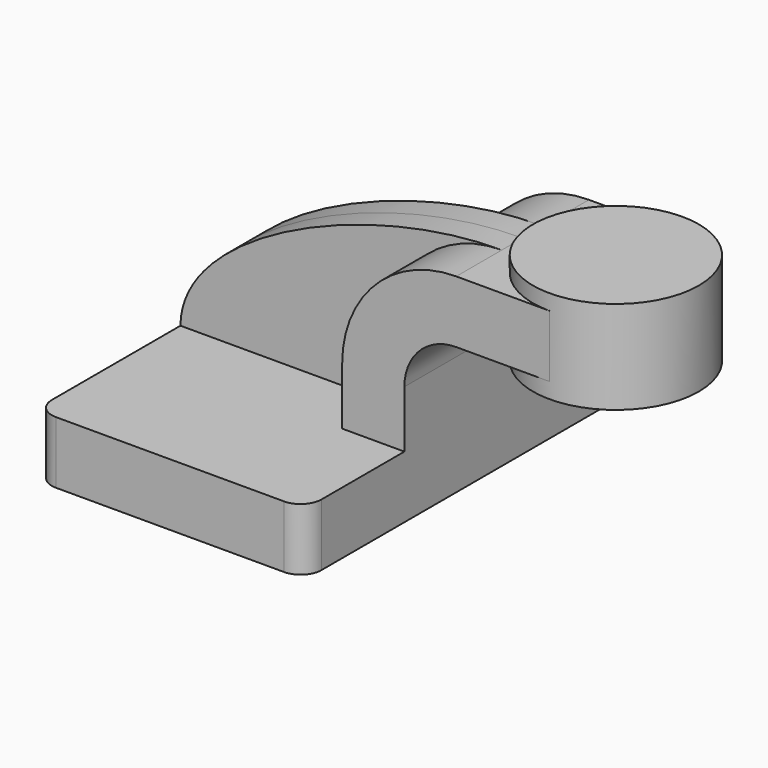
from build123d import *

# Parameters (mm, degrees)
F1_DEPTH = 63.5
F2_DEPTH = 25.4
F3_DEPTH = 7.9375
F0_W     = 25.4
F0_H     = 19.0500000358
F4_DEPTH = 25.4
F6_R     = 6.35


# Not quite as in the source:
# - a feature names something its author has since deleted; it is built from what else it names


with BuildPart() as f1:
    # F0 (on Front) → F1 (new body, symmetric)
    with BuildSketch(Plane.XZ):
        Polygon((-41.275, 9.525), (-41.275, -9.525), (41.275, -9.525), (41.275, 9.525), (22.2249999642, 9.525), align=None)
    extrude(amount=F1_DEPTH, both=True)

    # F0 (on Front) → F2 (join, symmetric)
    with BuildSketch(Plane.XZ):
        with BuildLine():
            Line((22.2249999642, 9.525), (41.275, 9.525))
            Line((41.275, 9.525), (41.275, 27.0002))
            ThreePointArc((41.275, 27.0002), (45.9246798487, 38.2255201513), (57.15, 42.8752))
            Line((57.15, 42.8752), (60.325, 42.8752))
            Line((60.325, 42.8752), (60.325, 61.9252000358))
            Line((60.325, 61.9252000358), (57.15, 61.9252000358))
            ThreePointArc((57.15, 61.9252000358), (32.4542956418, 51.6959043582), (22.2249999642, 27.0002))
            Line((22.2249999642, 27.0002), (22.2249999642, 9.525))
        make_face()
    extrude(amount=F2_DEPTH, both=True)

    # F0 (on Front) → F3 (join, symmetric)
    with BuildSketch(Plane.XZ):
        with BuildLine():
            add(Edge.make_bspline(
                [(-41.275, 9.525), (-41.1172062159, 36.9034484029), (15.5369872227, 62.0494298637), (57.15, 61.9252000358)],
                knots=[0, 0, 0, 0, 111.5045361803, 111.5045361803, 111.5045361803, 111.5045361803], degree=3))
            Line((-41.275, 9.525), (22.2249999642, 9.525))
            Line((22.2249999642, 9.525), (22.2249999642, 27.0002))
            ThreePointArc((22.2249999642, 27.0002), (32.4542956418, 51.6959043582), (57.15, 61.9252000358))
        make_face()
    extrude(amount=F3_DEPTH, both=True)

    # F0 (on Front) → F4 (join, symmetric)
    with BuildSketch(Plane.XZ):
        with Locations((73.025, 52.4002000179)):
            Rectangle(F0_W, F0_H)
    extrude(amount=F4_DEPTH, both=True)

    # F0 (on Front) → F5 (revolve)
    with BuildSketch(Plane.XZ):
        Polygon((85.725, 66.675), (85.725, 61.9252000358), (85.725, 42.8752), (85.725, 38.1), (111.125, 38.1), (111.125, 66.675), align=None)
    revolve(axis=Axis((85.725, 0, 52.3875), (0, 0, 1)))

    # F6
    f6_edges = [f1.edges().sort_by_distance(p)[0] for p in [
        (41.275, -63.5, 0),
        (-41.275, -63.5, 0),
        (41.275, 63.5, 0),
        (-41.275, 63.5, 0),
    ]]
    fillet(f6_edges, radius=F6_R)


solid = f1.part
